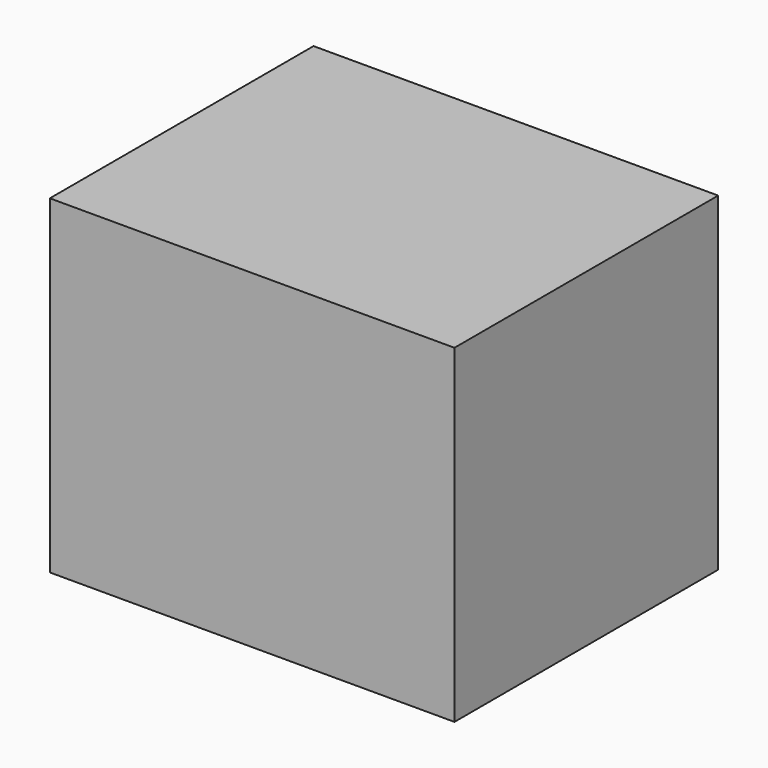
from build123d import *

# Parameters (mm, degrees)
F0_W     = 83.4715105593
F0_H     = 67.9460968822
F1_DEPTH = 68


# Not quite as in the source:
# - a feature of the source that left no trace in its solid (it failed there, or was rolled back) is left out


with BuildPart() as f1:
    # F0 (on Front) → F1 (new body)
    with BuildSketch(Plane.XZ):
        with Locations((3.5400893539, -7.3624784127)):
            Rectangle(F0_W, F0_H)
    extrude(amount=F1_DEPTH)


solid = f1.part
